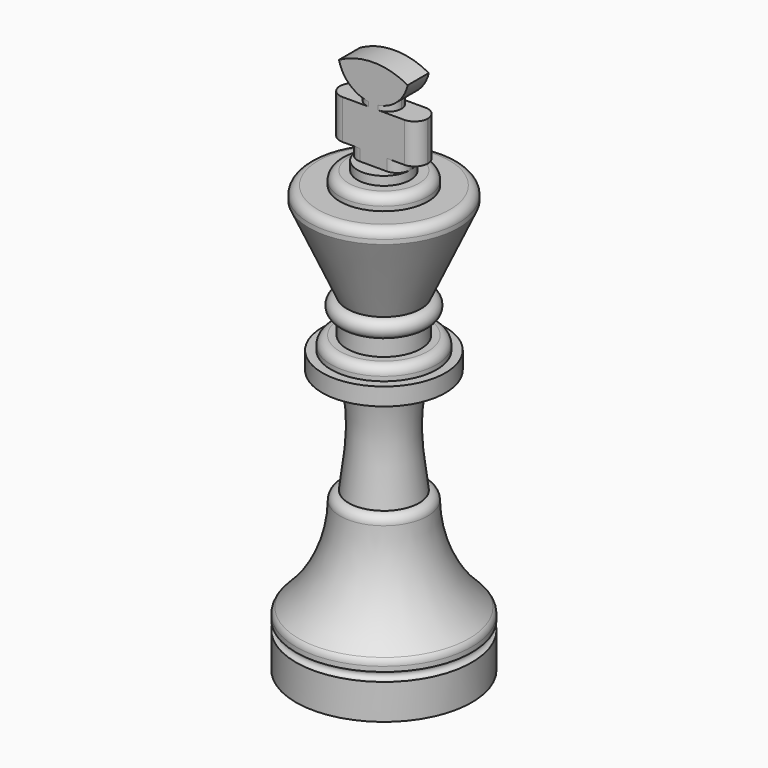
from build123d import *

# Parameters (mm, degrees)
F4_DEPTH     = 1.5
F5_T1_DEPTH  = 4.5
F5_T3_DEPTH  = 1.3
F5_T8_DEPTH  = 4.7524143468
F5_S9_R      = 4
F5_T10_DEPTH = 4
F5_T14_DEPTH = 4.7524143468
F5_S15_R     = 4
F5_T16_DEPTH = 4
F5_T20_DEPTH = 4.7524143468
F5_S21_R     = 4
F5_T22_DEPTH = 4
F5_T26_DEPTH = 4.7524143468
F5_S27_R     = 4
F5_T28_DEPTH = 4


# Not quite as in the source:
# - a fillet or chamfer that OpenCascade refuses, or shapes differently, is made with other operations: its cross-section is extruded or revolved along the edge and cut away or added


with BuildPart() as f1:
    # F0 (on Front) → F1 (revolve)
    with BuildSketch(Plane.XZ):
        with BuildLine():
            Line((-10, 0), (0, 0))
            Line((0, 0), (0, 51))
            Line((0, 51), (-3, 51))
            Line((-3, 51), (-3, 50))
            Line((-3, 50), (-5, 50))
            Line((-5, 50), (-5, 48.5))
            Line((-5, 48.5), (-8.5, 48.5))
            Line((-8.5, 48.5), (-8.5, 47))
            Line((-8.5, 47), (-4.2, 37.5))
            ThreePointArc((-4.2, 37.5), (-5.2, 36.5), (-4.2, 35.5))
            Line((-4.2, 35.5), (-4.2, 33.5))
            Line((-4.2, 33.5), (-6, 33.5))
            Line((-6, 33.5), (-6, 32))
            Line((-6, 32), (-7, 32))
            Line((-7, 32), (-7, 30))
            Line((-7, 30), (-4, 30))
            add(Edge.make_bspline(
                [(-4, 18), (-3.2570937183, 23.4906580299), (-3.0659101903, 25.0201262534), (-4, 30)],
                knots=[0, 0, 0, 0, 12, 12, 12, 12], degree=3))
            Line((-4, 18), (-5, 18))
            ThreePointArc((-5, 18), (-6.1324669242, 11.4301945518), (-10, 6))
            Line((-10, 6), (-10, 5))
            ThreePointArc((-10, 5), (-9.5, 4.5), (-10, 4))
            Line((-10, 4), (-10, 0))
        make_face()
    revolve(axis=Axis((0, 0, 25.5), (0, 0, -1)))

    # F2: fillet of radius 1 on 5 edges, made by hand

    # F2_s1 → F2_t2 (revolve, cut)
    with BuildSketch(Plane.XZ):
        with BuildLine():
            ThreePointArc((-9.6861637982, 6.2877192457), (-9.9181949135, 5.9564010683), (-10, 5.560272174))
            Line((-10, 5.560272174), (-10, 6))
            ThreePointArc((-10, 6), (-9.8420610087, 6.1427460638), (-9.6861637982, 6.2877192457))
        make_face()
    revolve(axis=Axis((0, 0, 6), (0, 0, -1)), mode=Mode.SUBTRACT)

    # F2_s3 → F2_t4 (revolve, cut)
    with BuildSketch(Plane.XZ):
        with BuildLine():
            ThreePointArc((-4.979783597, 17.0126542149), (-4.6896809685, 17.7045860706), (-4, 18))
            Line((-4, 18), (-5, 18))
            ThreePointArc((-5, 18), (-4.9817641292, 17.5064935256), (-4.979783597, 17.0126542149))
        make_face()
    revolve(axis=Axis((0, 0, 18), (0, 0, -1)), mode=Mode.SUBTRACT)

    # F2_s5 → F2_t6 (revolve, cut)
    with BuildSketch(Plane.XZ):
        with BuildLine():
            ThreePointArc((-5, 33.5), (-5.7071067812, 33.2071067812), (-6, 32.5))
            Line((-6, 32.5), (-6, 33.5))
            Line((-6, 33.5), (-5, 33.5))
        make_face()
    revolve(axis=Axis((0, 0, 33.5), (0, 0, -1)), mode=Mode.SUBTRACT)

    # F2_s7 → F2_t8 (revolve, cut)
    with BuildSketch(Plane.XZ):
        with BuildLine():
            ThreePointArc((-7.5, 48.5), (-8.2071067812, 48.2071067812), (-8.5, 47.5))
            Line((-8.5, 47.5), (-8.5, 48.5))
            Line((-8.5, 48.5), (-7.5, 48.5))
        make_face()
    revolve(axis=Axis((0, 0, 48.5), (0, 0, -1)), mode=Mode.SUBTRACT)

    # F2_s9 → F2_t10 (revolve, cut)
    with BuildSketch(Plane.XZ):
        with BuildLine():
            ThreePointArc((-4, 50), (-4.7071067812, 49.7071067812), (-5, 49))
            Line((-5, 49), (-5, 50))
            Line((-5, 50), (-4, 50))
        make_face()
    revolve(axis=Axis((0, 0, 50), (0, 0, -1)), mode=Mode.SUBTRACT)

    # F3 (on Front) → F4 (join, symmetric)
    with BuildSketch(Plane.XZ):
        with BuildLine():
            Line((-3, 51), (0, 51))
            Line((0, 51), (3, 51))
            Line((3, 51), (3, 52.3))
            Line((3, 52.3), (5, 52.3))
            Line((5, 52.3), (5, 56.8))
            Line((5, 56.8), (2, 56.8))
            Line((2, 56.8), (2, 57.8))
            ThreePointArc((2, 57.8), (3.2237742518, 58.8961321107), (3.903712088, 60.3917301725))
            ThreePointArc((3.903712088, 60.3917301725), (0, 61.4088201821), (-3.903712088, 60.3917301725))
            ThreePointArc((-3.903712088, 60.3917301725), (-3.2237742518, 58.8961321107), (-2, 57.8))
            Line((-2, 57.8), (-2, 56.8))
            Line((-2, 56.8), (-5, 56.8))
            Line((-5, 56.8), (-5, 52.3))
            Line((-5, 52.3), (-3, 52.3))
            Line((-3, 52.3), (-3, 51))
        make_face()
    extrude(amount=F4_DEPTH, both=True)

    # F5: fillet of radius 1.5 on 12 edges, made by hand

    # F5_s2 → F5_t1 (cut)
    with BuildSketch(Plane.XY.offset(52.3)):
        with BuildLine():
            ThreePointArc((-3.4990343146, -1.5004), (-4.5606601718, -1.0606601718), (-5.0004, 0.0009656854))
            Line((-5.0004, 0.0009656854), (-5.1505365685, 0.0009656854))
            ThreePointArc((-5.1505365685, 0.0009656854), (-5.1501365685, -0.7495171573), (-5.1501365685, -1.5))
            Line((-5.1501365685, -1.5), (-5, -1.6501365685))
            ThreePointArc((-5, -1.6501365685), (-4.2495171573, -1.6501365685), (-3.4990343146, -1.6505365685))
            Line((-3.4990343146, -1.6505365685), (-3.4990343146, -1.5004))
        make_face()
        with BuildLine():
            ThreePointArc((-3.4990343146, 1.5004), (-4.5606601718, 1.0606601718), (-5.0004, -0.0009656854))
            Line((-5.0004, -0.0009656854), (-5.1505365685, -0.0009656854))
            ThreePointArc((-5.1505365685, -0.0009656854), (-5.1501365685, 0.7495171573), (-5.1501365685, 1.5))
            Line((-5.1501365685, 1.5), (-5, 1.6501365685))
            ThreePointArc((-5, 1.6501365685), (-4.2495171573, 1.6501365685), (-3.4990343146, 1.6505365685))
            Line((-3.4990343146, 1.6505365685), (-3.4990343146, 1.5004))
        make_face()
        with BuildLine():
            ThreePointArc((3.4990343146, -1.5004), (4.5606601718, -1.0606601718), (5.0004, 0.0009656854))
            Line((5.0004, 0.0009656854), (5.1505365685, 0.0009656854))
            ThreePointArc((5.1505365685, 0.0009656854), (5.1501365685, -0.7495171573), (5.1501365685, -1.5))
            Line((5.1501365685, -1.5), (5, -1.6501365685))
            ThreePointArc((5, -1.6501365685), (4.2495171573, -1.6501365685), (3.4990343146, -1.6505365685))
            Line((3.4990343146, -1.6505365685), (3.4990343146, -1.5004))
        make_face()
        with BuildLine():
            ThreePointArc((3.4990343146, 1.5004), (4.5606601718, 1.0606601718), (5.0004, -0.0009656854))
            Line((5.0004, -0.0009656854), (5.1505365685, -0.0009656854))
            ThreePointArc((5.1505365685, -0.0009656854), (5.1501365685, 0.7495171573), (5.1501365685, 1.5))
            Line((5.1501365685, 1.5), (5, 1.6501365685))
            ThreePointArc((5, 1.6501365685), (4.2495171573, 1.6501365685), (3.4990343146, 1.6505365685))
            Line((3.4990343146, 1.6505365685), (3.4990343146, 1.5004))
        make_face()
    extrude(amount=F5_T1_DEPTH, mode=Mode.SUBTRACT)

    # F5_s4 → F5_t3 (cut)
    with BuildSketch(Plane.XY.offset(51)):
        with BuildLine():
            ThreePointArc((3.0004, -0.0009656854), (2.5606601718, 1.0606601718), (1.4990343146, 1.5004))
            Line((1.4990343146, 1.5004), (1.4990343146, 1.6505365685))
            ThreePointArc((1.4990343146, 1.6505365685), (2.2495171573, 1.6501365685), (3, 1.6501365685))
            Line((3, 1.6501365685), (3.1501365685, 1.5))
            ThreePointArc((3.1501365685, 1.5), (3.1501365685, 0.7495171573), (3.1505365685, -0.0009656854))
            Line((3.1505365685, -0.0009656854), (3.0004, -0.0009656854))
        make_face()
        with BuildLine():
            ThreePointArc((1.4990343146, -1.5004), (2.5606601718, -1.0606601718), (3.0004, 0.0009656854))
            Line((3.0004, 0.0009656854), (3.1505365685, 0.0009656854))
            ThreePointArc((3.1505365685, 0.0009656854), (3.1501365685, -0.7495171573), (3.1501365685, -1.5))
            Line((3.1501365685, -1.5), (3, -1.6501365685))
            ThreePointArc((3, -1.6501365685), (2.2495171573, -1.6501365685), (1.4990343146, -1.6505365685))
            Line((1.4990343146, -1.6505365685), (1.4990343146, -1.5004))
        make_face()
        with BuildLine():
            ThreePointArc((-3.0004, 0.0009656854), (-2.5606601718, -1.0606601718), (-1.4990343146, -1.5004))
            Line((-1.4990343146, -1.5004), (-1.4990343146, -1.6505365685))
            ThreePointArc((-1.4990343146, -1.6505365685), (-2.2495171573, -1.6501365685), (-3, -1.6501365685))
            Line((-3, -1.6501365685), (-3.1501365685, -1.5))
            ThreePointArc((-3.1501365685, -1.5), (-3.1501365685, -0.7495171573), (-3.1505365685, 0.0009656854))
            Line((-3.1505365685, 0.0009656854), (-3.0004, 0.0009656854))
        make_face()
        with BuildLine():
            ThreePointArc((-3.0004, -0.0009656854), (-2.5606601718, 1.0606601718), (-1.4990343146, 1.5004))
            Line((-1.4990343146, 1.5004), (-1.4990343146, 1.6505365685))
            ThreePointArc((-1.4990343146, 1.6505365685), (-2.2495171573, 1.6501365685), (-3, 1.6501365685))
            Line((-3, 1.6501365685), (-3.1501365685, 1.5))
            ThreePointArc((-3.1501365685, 1.5), (-3.1501365685, 0.7495171573), (-3.1505365685, -0.0009656854))
            Line((-3.1505365685, -0.0009656854), (-3.0004, -0.0009656854))
        make_face()
    extrude(amount=F5_T3_DEPTH, mode=Mode.SUBTRACT)


with BuildPart() as f5_tool6:
    # F5_s7 → F5_t8 (new body)
    with BuildSketch(Plane.XY.offset(61.5524143468)):
        with BuildLine():
            ThreePointArc((-0.4990343146, -1.5004), (-1.5606601718, -1.0606601718), (-2.0004, 0.0009656854))
            Line((-2.0004, 0.0009656854), (-2.1505365685, 0.0009656854))
            ThreePointArc((-2.1505365685, 0.0009656854), (-2.1501365685, -0.7495171573), (-2.1501365685, -1.5))
            Line((-2.1501365685, -1.5), (-2, -1.6501365685))
            ThreePointArc((-2, -1.6501365685), (-1.2495171573, -1.6501365685), (-0.4990343146, -1.6505365685))
            Line((-0.4990343146, -1.6505365685), (-0.4990343146, -1.5004))
        make_face()
    extrude(amount=-F5_T8_DEPTH)

    # F5_s9 → F5_t10 (cut, symmetric)
    with BuildSketch(Plane.XZ.offset(0.8)):
        with Locations((0, 61.2641016151)):
            Circle(F5_S9_R)
    extrude(amount=F5_T10_DEPTH, both=True, mode=Mode.SUBTRACT)


with BuildPart() as f1_1:
    add(f1.part)

    # F5_t5: cut F5_tool6
    add(f5_tool6.part, mode=Mode.SUBTRACT)


with BuildPart() as f5_tool12:
    # F5_s13 → F5_t14 (new body)
    with BuildSketch(Plane.XY.offset(56.8)):
        with BuildLine():
            ThreePointArc((0.4990343146, -1.5004), (1.5606601718, -1.0606601718), (2.0004, 0.0009656854))
            Line((2.0004, 0.0009656854), (2.1505365685, 0.0009656854))
            ThreePointArc((2.1505365685, 0.0009656854), (2.1501365685, -0.7495171573), (2.1501365685, -1.5))
            Line((2.1501365685, -1.5), (2, -1.6501365685))
            ThreePointArc((2, -1.6501365685), (1.2495171573, -1.6501365685), (0.4990343146, -1.6505365685))
            Line((0.4990343146, -1.6505365685), (0.4990343146, -1.5004))
        make_face()
    extrude(amount=F5_T14_DEPTH)

    # F5_s15 → F5_t16 (cut, symmetric)
    with BuildSketch(Plane.XZ.offset(0.8)):
        with Locations((0, 61.2641016151)):
            Circle(F5_S15_R)
    extrude(amount=F5_T16_DEPTH, both=True, mode=Mode.SUBTRACT)


with BuildPart() as f1_2:
    add(f1_1.part)

    # F5_t11: cut F5_tool12
    add(f5_tool12.part, mode=Mode.SUBTRACT)


with BuildPart() as f5_tool18:
    # F5_s19 → F5_t20 (new body)
    with BuildSketch(Plane.XY.offset(61.5524143468)):
        with BuildLine():
            ThreePointArc((-0.4990343146, 1.5004), (-1.5606601718, 1.0606601718), (-2.0004, -0.0009656854))
            Line((-2.0004, -0.0009656854), (-2.1505365685, -0.0009656854))
            ThreePointArc((-2.1505365685, -0.0009656854), (-2.1501365685, 0.7495171573), (-2.1501365685, 1.5))
            Line((-2.1501365685, 1.5), (-2, 1.6501365685))
            ThreePointArc((-2, 1.6501365685), (-1.2495171573, 1.6501365685), (-0.4990343146, 1.6505365685))
            Line((-0.4990343146, 1.6505365685), (-0.4990343146, 1.5004))
        make_face()
    extrude(amount=-F5_T20_DEPTH)

    # F5_s21 → F5_t22 (cut, symmetric)
    with BuildSketch(Plane.XZ.offset(-0.8)):
        with Locations((0, 61.2641016151)):
            Circle(F5_S21_R)
    extrude(amount=F5_T22_DEPTH, both=True, mode=Mode.SUBTRACT)


with BuildPart() as f1_3:
    add(f1_2.part)

    # F5_t17: cut F5_tool18
    add(f5_tool18.part, mode=Mode.SUBTRACT)


with BuildPart() as f5_tool24:
    # F5_s25 → F5_t26 (new body)
    with BuildSketch(Plane.XY.offset(56.8)):
        with BuildLine():
            ThreePointArc((0.4990343146, 1.5004), (1.5606601718, 1.0606601718), (2.0004, -0.0009656854))
            Line((2.0004, -0.0009656854), (2.1505365685, -0.0009656854))
            ThreePointArc((2.1505365685, -0.0009656854), (2.1501365685, 0.7495171573), (2.1501365685, 1.5))
            Line((2.1501365685, 1.5), (2, 1.6501365685))
            ThreePointArc((2, 1.6501365685), (1.2495171573, 1.6501365685), (0.4990343146, 1.6505365685))
            Line((0.4990343146, 1.6505365685), (0.4990343146, 1.5004))
        make_face()
    extrude(amount=F5_T26_DEPTH)

    # F5_s27 → F5_t28 (cut, symmetric)
    with BuildSketch(Plane.XZ.offset(-0.8)):
        with Locations((0, 61.2641016151)):
            Circle(F5_S27_R)
    extrude(amount=F5_T28_DEPTH, both=True, mode=Mode.SUBTRACT)


with BuildPart() as f1_4:
    add(f1_3.part)

    # F5_t23: cut F5_tool24
    add(f5_tool24.part, mode=Mode.SUBTRACT)


solid = f1_4.part
